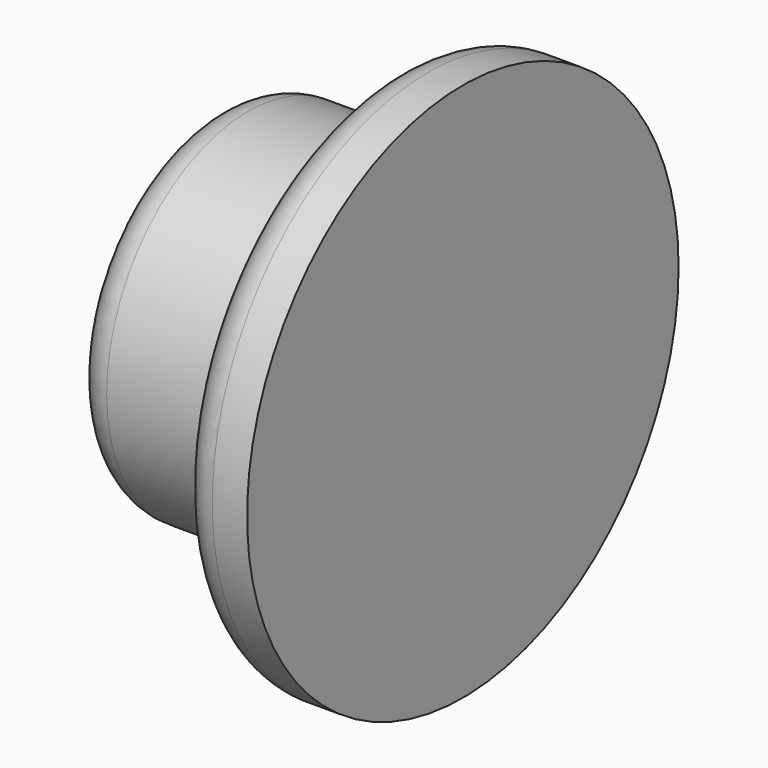
from build123d import *

# Parameters (mm, degrees)
F0_R     = 25
F0_R_2   = 20
F1_DEPTH = 25.4
F2_R     = 38.1
F2_R_2   = 25
F2_R_3   = 20
F3_DEPTH = 10


# Not quite as in the source:
# - a fillet or chamfer that OpenCascade refuses, or shapes differently, is made with other operations: its cross-section is extruded or revolved along the edge and cut away or added


with BuildPart() as f1:
    # F0 (on Right) → F1 (new body)
    with BuildSketch(Plane.YZ):
        Circle(F0_R)
        Circle(F0_R_2, mode=Mode.SUBTRACT)
    extrude(amount=F1_DEPTH)

    # F2 (on face) → F3 (join)
    with BuildSketch(Plane.YZ.offset(25.4)):
        Circle(F2_R)
        Circle(F2_R_2, mode=Mode.SUBTRACT)
        Circle(F2_R_2)
        Circle(F2_R_3, mode=Mode.SUBTRACT)
        Circle(F2_R_3)
    extrude(amount=F3_DEPTH)

    # F4: fillet of radius 5.08 on 4 edges, made by hand

    # F4_s1 → F4_t2 (revolve)
    with BuildSketch(Plane.XY):
        with BuildLine():
            ThreePointArc((25.4, 30.08), (23.9121024484, 26.4878975516), (20.32, 25))
            Line((20.32, 25), (25.4, 25))
            Line((25.4, 25), (25.4, 30.08))
        make_face()
    revolve(axis=Axis((25.4, 0, 0), (1, 0, 0)))

    # F4_s3 → F4_t4 (revolve, cut)
    with BuildSketch(Plane.XY):
        with BuildLine():
            ThreePointArc((5.08, 25), (1.4878975516, 23.5121024484), (0, 19.92))
            Line((0, 19.92), (0, 25))
            Line((0, 25), (5.08, 25))
        make_face()
    revolve(axis=Axis((0, 0, 0), (1, 0, 0)), mode=Mode.SUBTRACT)

    # F4_s5 → F4_t6 (revolve, cut)
    with BuildSketch(Plane.XY):
        with BuildLine():
            ThreePointArc((30.48, 38.1), (26.8878975516, 36.6121024484), (25.4, 33.02))
            Line((25.4, 33.02), (25.4, 38.1))
            Line((25.4, 38.1), (30.48, 38.1))
        make_face()
    revolve(axis=Axis((25.4, 0, 0), (1, 0, 0)), mode=Mode.SUBTRACT)

    # F5: chamfer of 1.524 on 1 edges, made by hand

    # F5_s1 → F5_t2 (revolve, cut)
    with BuildSketch(Plane.XY):
        with BuildLine():
            Line((0.4894859208, 22.2141433772), (1.9000393506, 19.9482483046))
            Line((1.9000393506, 19.9482483046), (1.9000393506, 19.9177683046))
            ThreePointArc((1.9000393506, 19.9177683046), (0.9503346555, 19.96952), (0.0006299603, 19.96952))
            Line((0.0006299603, 19.96952), (-0.0298462599, 20.00048))
            ThreePointArc((-0.0298462599, 20.00048), (0.1169178679, 21.1385325522), (0.4621361335, 22.2275977273))
            Line((0.4621361335, 22.2275977273), (0.4894859208, 22.2141433772))
        make_face()
    revolve(axis=Axis((0.0006299603, 0, 0), (-1, 0, 0)), mode=Mode.SUBTRACT)


solid = f1.part
